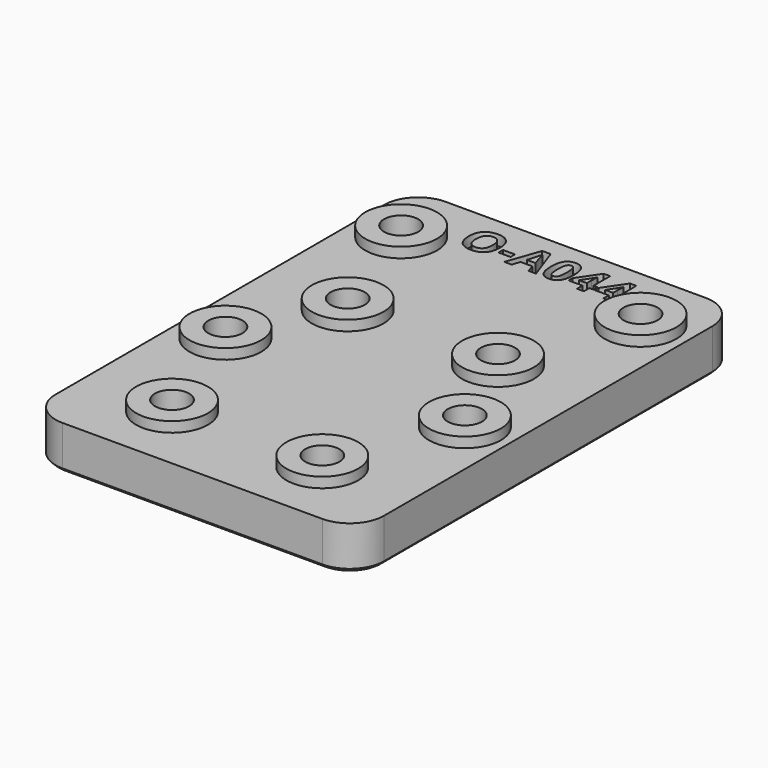
from build123d import *

# Parameters (mm, degrees)
F0_W         = 48
F0_H         = 70
F0_R         = 2.5
F1_DEPTH     = 6.35
F2_R         = 5
F3_TEXT_SIZE = 6.7241605744
F4_DEPTH     = 1.5
F5_SIZE      = 0.5
F6_R         = 5.25
F6_R_2       = 2.5
F7_DEPTH     = 1.5


# Not quite as in the source:
# - Text() gives the source's letters only with a copy of the font that has no kerning and outlines rounded to 1/6400 em; it was checked with that copy


with BuildPart() as f1:
    # F0 (on Top) → F1 (new body)
    with BuildSketch(Plane.XY):
        Rectangle(F0_W, F0_H)
        with Locations((-10.9845162696, -25)):
            Circle(F0_R, mode=Mode.SUBTRACT)
        with Locations((-17.5, -7.098855574)):
            Circle(F0_R, mode=Mode.SUBTRACT)
        with Locations((10.9845162696, -25)):
            Circle(F0_R, mode=Mode.SUBTRACT)
        with Locations((17.5, -7.098855574)):
            Circle(F0_R, mode=Mode.SUBTRACT)
        with Locations((-10.9845162696, 7.098855574)):
            Circle(F0_R, mode=Mode.SUBTRACT)
        with Locations((-17.5, 25)):
            Circle(F0_R, mode=Mode.SUBTRACT)
        with Locations((10.9845162696, 7.098855574)):
            Circle(F0_R, mode=Mode.SUBTRACT)
        with Locations((17.5, 25)):
            Circle(F0_R, mode=Mode.SUBTRACT)
    extrude(amount=F1_DEPTH)

    # F2
    f2_edges = [f1.edges().sort_by_distance(p)[0] for p in [
        (-24, 35, 3.175),
        (24, 35, 3.175),
        (-24, -35, 3.175),
        (24, -35, 3.175),
    ]]
    fillet(f2_edges, radius=F2_R)

    # F3 (on face) → F4 (cut)
    with BuildSketch(Plane.XY.offset(6.35)):
        with Locations((-12, 27.5793021932)):
            Text('O-A044', F3_TEXT_SIZE, font='Open Sans', font_style=FontStyle.BOLD, text_align=(TextAlign.LEFT, TextAlign.BOTTOM))
    extrude(amount=-F4_DEPTH, mode=Mode.SUBTRACT)

    # F5
    f5_edges = [f1.edges().sort_by_distance(p)[0] for p in [
        (0, -35, 0),
    ]]
    chamfer(f5_edges, length=F5_SIZE)

    # F6 (on face) → F7 (join)
    with BuildSketch(Plane.XY.offset(6.35)):
        with Locations((-17.5, 25)):
            Circle(F6_R)
        with Locations((-17.5, 25)):
            Circle(F6_R_2, mode=Mode.SUBTRACT)
        with Locations((-10.9845162696, 7.098855574)):
            Circle(F6_R)
        with Locations((-10.9845162696, 7.098855574)):
            Circle(F6_R_2, mode=Mode.SUBTRACT)
        with Locations((17.5, 25)):
            Circle(F6_R)
        with Locations((17.5, 25)):
            Circle(F6_R_2, mode=Mode.SUBTRACT)
        with Locations((10.9845162696, 7.098855574)):
            Circle(F6_R)
        with Locations((10.9845162696, 7.098855574)):
            Circle(F6_R_2, mode=Mode.SUBTRACT)
        with Locations((17.5, -7.098855574)):
            Circle(F6_R)
        with Locations((17.5, -7.098855574)):
            Circle(F6_R_2, mode=Mode.SUBTRACT)
        with Locations((10.9845162696, -25)):
            Circle(F6_R)
        with Locations((10.9845162696, -25)):
            Circle(F6_R_2, mode=Mode.SUBTRACT)
        with Locations((-10.9845162696, -25)):
            Circle(F6_R)
        with Locations((-10.9845162696, -25)):
            Circle(F6_R_2, mode=Mode.SUBTRACT)
        with Locations((-17.5, -7.098855574)):
            Circle(F6_R)
        with Locations((-17.5, -7.098855574)):
            Circle(F6_R_2, mode=Mode.SUBTRACT)
    extrude(amount=F7_DEPTH)


solid = f1.part
